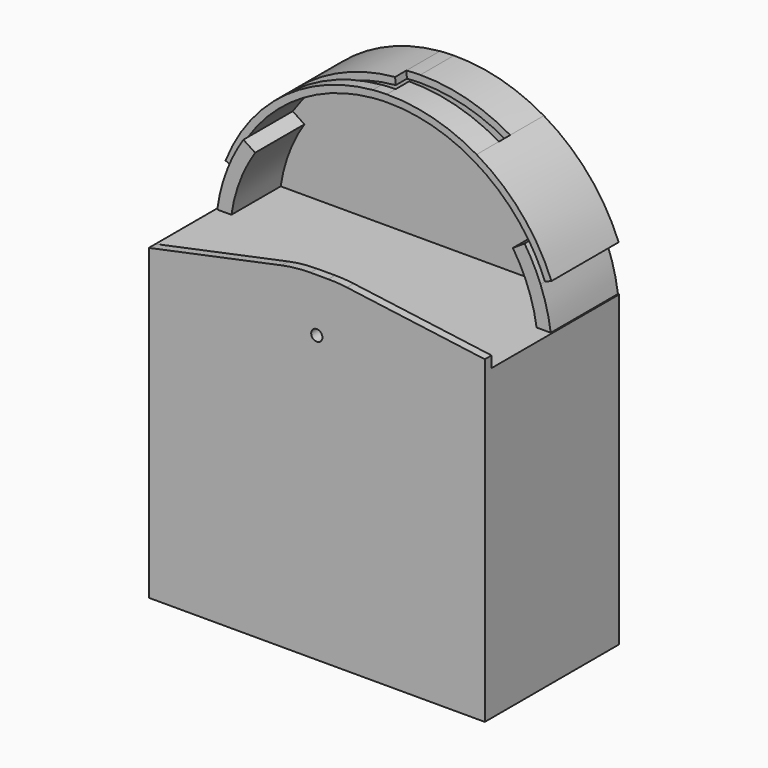
from build123d import *

# Parameters (mm, degrees)
F1_DEPTH      = 60
F2_DEPTH      = 60
F3_DEPTH      = 8
F4_DEPTH      = 30
F5_DEPTH      = 28
F5_DEPTH_BACK = 2
F6_START      = 13
F6_DEPTH      = 5
F7_START      = 18
F7_DEPTH      = 6
F8_D          = 4
F11_DEPTH     = 3


with BuildPart() as f1:
    # F0 (on Front) → F1 (new body)
    with BuildSketch(Plane.XZ):
        Polygon((-54.993186, 3), (-60, 3), (-60, -102), (60, -102), (60, 3), (54.993186, 3), align=None)
    extrude(amount=F1_DEPTH)

    # F0 (on Front) → F2 (join)
    with BuildSketch(Plane.XZ):
        with BuildLine():
            Line((54.490829, 8), (-54.490829, 8))
            ThreePointArc((-54.490829, 8), (-54.799064, 5.505733), (-54.993186, 3))
            Line((-54.993186, 3), (54.993186, 3))
            ThreePointArc((54.993186, 3), (54.799064, 5.505733), (54.490829, 8))
        make_face()
        with BuildLine():
            Line((-59.539903, 8), (-60, 8))
            Line((-60, 8), (-60, 3))
            ThreePointArc((-60, 3), (-59.822212, 5.504809), (-59.539903, 8))
        make_face()
        with BuildLine():
            Line((60, 8), (59.539903, 8))
            ThreePointArc((59.539903, 8), (59.822212, 5.504809), (60, 3))
            Line((60, 3), (60, 8))
        make_face()
        with BuildLine():
            Line((-54.490829, 8), (-59.539903, 8))
            ThreePointArc((-59.539903, 8), (-59.822212, 5.504809), (-60, 3))
            Line((-60, 3), (-54.993186, 3))
            ThreePointArc((-54.993186, 3), (-54.799064, 5.505733), (-54.490829, 8))
        make_face()
        with BuildLine():
            Line((59.539903, 8), (54.490829, 8))
            ThreePointArc((54.490829, 8), (54.799064, 5.505733), (54.993186, 3))
            Line((54.993186, 3), (60, 3))
            ThreePointArc((60, 3), (59.822212, 5.504809), (59.539903, 8))
        make_face()
    extrude(amount=F2_DEPTH)

    # F0 (on Front) → F3 (join)
    with BuildSketch(Plane.XZ):
        with BuildLine():
            Line((54.490829, 8), (-54.490829, 8))
            ThreePointArc((-54.490829, 8), (-54.799064, 5.505733), (-54.993186, 3))
            Line((-54.993186, 3), (54.993186, 3))
            ThreePointArc((54.993186, 3), (54.799064, 5.505733), (54.490829, 8))
        make_face()
        with BuildLine():
            Line((-59.539903, 8), (-60, 8))
            Line((-60, 8), (-60, 3))
            ThreePointArc((-60, 3), (-59.822212, 5.504809), (-59.539903, 8))
        make_face()
        with BuildLine():
            ThreePointArc((-46.021521, 30.253431), (-51.473167, 19.589884), (-54.490829, 8))
            Line((-54.490829, 8), (54.490829, 8))
            ThreePointArc((54.490829, 8), (51.473167, 19.589884), (46.021521, 30.253431))
            ThreePointArc((46.021521, 30.253431), (0, 55.074953), (-46.021521, 30.253431))
        make_face()
        with BuildLine():
            ThreePointArc((46.021521, 30.253431), (51.473167, 19.589884), (54.490829, 8))
            Line((54.490829, 8), (59.539903, 8))
            ThreePointArc((59.539903, 8), (58.13273, 15.152087), (55.869714, 22.081102))
            ThreePointArc((55.869714, 22.081102), (53.314918, 27.686088), (50.199602, 33))
            Line((50.199602, 33), (46.021521, 30.253431))
        make_face()
        with BuildLine():
            Line((-50.199602, 33), (-46.021521, 30.253431))
            ThreePointArc((-46.021521, 30.253431), (0, 55.074953), (46.021521, 30.253431))
            Line((46.021521, 30.253431), (50.199602, 33))
            ThreePointArc((50.199602, 33), (41.302524, 43.624552), (30.207691, 51.92779))
            ThreePointArc((30.207691, 51.92779), (15.350043, 58.080773), (-0.607537, 60.071881))
            ThreePointArc((-0.607537, 60.071881), (-3.010066, 59.999496), (-5.407777, 59.831062))
            ThreePointArc((-5.407777, 59.831062), (-23.441919, 55.312534), (-39.230941, 45.496519))
            ThreePointArc((-39.230941, 45.496519), (-45.149709, 39.629582), (-50.199602, 33))
        make_face()
        with BuildLine():
            ThreePointArc((-55.869714, 22.081102), (-58.13273, 15.152087), (-59.539903, 8))
            Line((-59.539903, 8), (-54.490829, 8))
            ThreePointArc((-54.490829, 8), (-51.473167, 19.589884), (-46.021521, 30.253431))
            Line((-46.021521, 30.253431), (-50.199602, 33))
            ThreePointArc((-50.199602, 33), (-53.314918, 27.686088), (-55.869714, 22.081102))
        make_face()
        with BuildLine():
            Line((-54.490829, 8), (-59.539903, 8))
            ThreePointArc((-59.539903, 8), (-59.822212, 5.504809), (-60, 3))
            Line((-60, 3), (-54.993186, 3))
            ThreePointArc((-54.993186, 3), (-54.799064, 5.505733), (-54.490829, 8))
        make_face()
        with BuildLine():
            Line((59.539903, 8), (54.490829, 8))
            ThreePointArc((54.490829, 8), (54.799064, 5.505733), (54.993186, 3))
            Line((54.993186, 3), (60, 3))
            ThreePointArc((60, 3), (59.822212, 5.504809), (59.539903, 8))
        make_face()
    extrude(amount=F3_DEPTH)

    # F0 (on Front) → F4 (join)
    with BuildSketch(Plane.XZ):
        with BuildLine():
            ThreePointArc((-55.869714, 22.081102), (-58.13273, 15.152087), (-59.539903, 8))
            Line((-59.539903, 8), (-54.490829, 8))
            ThreePointArc((-54.490829, 8), (-51.473167, 19.589884), (-46.021521, 30.253431))
            Line((-46.021521, 30.253431), (-50.199602, 33))
            ThreePointArc((-50.199602, 33), (-53.314918, 27.686088), (-55.869714, 22.081102))
        make_face()
        with BuildLine():
            ThreePointArc((46.021521, 30.253431), (51.473167, 19.589884), (54.490829, 8))
            Line((54.490829, 8), (59.539903, 8))
            ThreePointArc((59.539903, 8), (58.13273, 15.152087), (55.869714, 22.081102))
            ThreePointArc((55.869714, 22.081102), (53.314918, 27.686088), (50.199602, 33))
            Line((50.199602, 33), (46.021521, 30.253431))
        make_face()
        with BuildLine():
            Line((-59.539903, 8), (-60, 8))
            Line((-60, 8), (-60, 3))
            ThreePointArc((-60, 3), (-59.822212, 5.504809), (-59.539903, 8))
        make_face()
        with BuildLine():
            Line((-54.490829, 8), (-59.539903, 8))
            ThreePointArc((-59.539903, 8), (-59.822212, 5.504809), (-60, 3))
            Line((-60, 3), (-54.993186, 3))
            ThreePointArc((-54.993186, 3), (-54.799064, 5.505733), (-54.490829, 8))
        make_face()
        with BuildLine():
            Line((59.539903, 8), (54.490829, 8))
            ThreePointArc((54.490829, 8), (54.799064, 5.505733), (54.993186, 3))
            Line((54.993186, 3), (60, 3))
            ThreePointArc((60, 3), (59.822212, 5.504809), (59.539903, 8))
        make_face()
    extrude(amount=F4_DEPTH)

    # F8 (through all)
    with Locations(Plane(origin=(0, 0, 0), x_dir=(1, 0, 0), z_dir=(0, 1, 0))):
        with Locations((0, 0)):
            Hole(F8_D / 2)

    # F10 (on face) → F11 (join)
    with BuildSketch(Plane.XZ.offset(60)):
        with BuildLine():
            Line((-12.532776, 17.938755), (-60, 8))
            Line((-60, 8), (60, 8))
            Line((60, 8), (60, 12))
            Line((60, 12), (10.751658, 18.561983))
            ThreePointArc((10.751658, 18.561983), (7.457027, 18.890376), (4.147885, 19))
            Line((4.147885, 19), (-2.285909, 19))
            ThreePointArc((-2.285909, 19), (-7.436747, 18.733981), (-12.532776, 17.938755))
        make_face()
    extrude(amount=-F11_DEPTH)


with BuildPart() as f5:
    # F0 (on Front) → F5 (new body, two sides)
    with BuildSketch(Plane.XZ) as f5_sk:
        with BuildLine():
            Line((-58.194714, 23), (-55.869714, 22.081102))
            ThreePointArc((-55.869714, 22.081102), (-53.314918, 27.686088), (-50.199602, 33))
            ThreePointArc((-50.199602, 33), (-45.149709, 39.629582), (-39.230941, 45.496519))
            Line((-39.230941, 45.496519), (-40.863524, 47.389842))
            ThreePointArc((-40.863524, 47.389842), (-51.00833, 36.246034), (-58.194714, 23))
        make_face()
        with BuildLine():
            Line((-40.863524, 47.389842), (-39.230941, 45.496519))
            ThreePointArc((-39.230941, 45.496519), (-23.441919, 55.312534), (-5.407777, 59.831062))
            Line((-5.407777, 59.831062), (-5.63282, 62.320912))
            ThreePointArc((-5.63282, 62.320912), (-24.417447, 57.614348), (-40.863524, 47.389842))
        make_face()
        with BuildLine():
            Line((-5.63282, 62.320912), (-5.407777, 59.831062))
            ThreePointArc((-5.407777, 59.831062), (-3.010066, 59.999496), (-0.607537, 60.071881))
            Line((-0.607537, 60.071881), (-0.63282, 62.571753))
            ThreePointArc((-0.63282, 62.571753), (-3.135329, 62.496356), (-5.63282, 62.320912))
        make_face()
        with BuildLine():
            ThreePointArc((-0.607537, 60.071881), (15.350043, 58.080773), (30.207691, 51.92779))
            Line((30.207691, 51.92779), (31.464774, 54.088749))
            ThreePointArc((31.464774, 54.088749), (15.98883, 60.497786), (-0.63282, 62.571753))
            Line((-0.63282, 62.571753), (-0.607537, 60.071881))
        make_face()
        with BuildLine():
            ThreePointArc((50.199602, 33), (53.314918, 27.686088), (55.869714, 22.081102))
            Line((55.869714, 22.081102), (58.194714, 23))
            ThreePointArc((58.194714, 23), (47.44822, 40.795726), (31.464774, 54.088749))
            Line((31.464774, 54.088749), (30.207691, 51.92779))
            ThreePointArc((30.207691, 51.92779), (41.302524, 43.624552), (50.199602, 33))
        make_face()
    extrude(amount=F5_DEPTH)
    extrude(f5_sk.sketch, amount=-F5_DEPTH_BACK)

    # F0 (on Front) → F6 (cut)
    with BuildSketch(Plane.XZ.offset(F6_START)):
        with BuildLine():
            ThreePointArc((-0.607537, 60.071881), (15.350043, 58.080773), (30.207691, 51.92779))
            Line((30.207691, 51.92779), (31.464774, 54.088749))
            ThreePointArc((31.464774, 54.088749), (15.98883, 60.497786), (-0.63282, 62.571753))
            Line((-0.63282, 62.571753), (-0.607537, 60.071881))
        make_face()
        with BuildLine():
            Line((-5.63282, 62.320912), (-5.407777, 59.831062))
            ThreePointArc((-5.407777, 59.831062), (-3.010066, 59.999496), (-0.607537, 60.071881))
            Line((-0.607537, 60.071881), (-0.63282, 62.571753))
            ThreePointArc((-0.63282, 62.571753), (-3.135329, 62.496356), (-5.63282, 62.320912))
        make_face()
    extrude(amount=F6_DEPTH, mode=Mode.SUBTRACT)

    # F0 (on Front) → F7 (cut)
    with BuildSketch(Plane.XZ.offset(F7_START)):
        with BuildLine():
            Line((-5.63282, 62.320912), (-5.407777, 59.831062))
            ThreePointArc((-5.407777, 59.831062), (-3.010066, 59.999496), (-0.607537, 60.071881))
            Line((-0.607537, 60.071881), (-0.63282, 62.571753))
            ThreePointArc((-0.63282, 62.571753), (-3.135329, 62.496356), (-5.63282, 62.320912))
        make_face()
        with BuildLine():
            Line((-40.863524, 47.389842), (-39.230941, 45.496519))
            ThreePointArc((-39.230941, 45.496519), (-23.441919, 55.312534), (-5.407777, 59.831062))
            Line((-5.407777, 59.831062), (-5.63282, 62.320912))
            ThreePointArc((-5.63282, 62.320912), (-24.417447, 57.614348), (-40.863524, 47.389842))
        make_face()
    extrude(amount=F7_DEPTH, mode=Mode.SUBTRACT)


solid = Compound([f1.part, f5.part])
